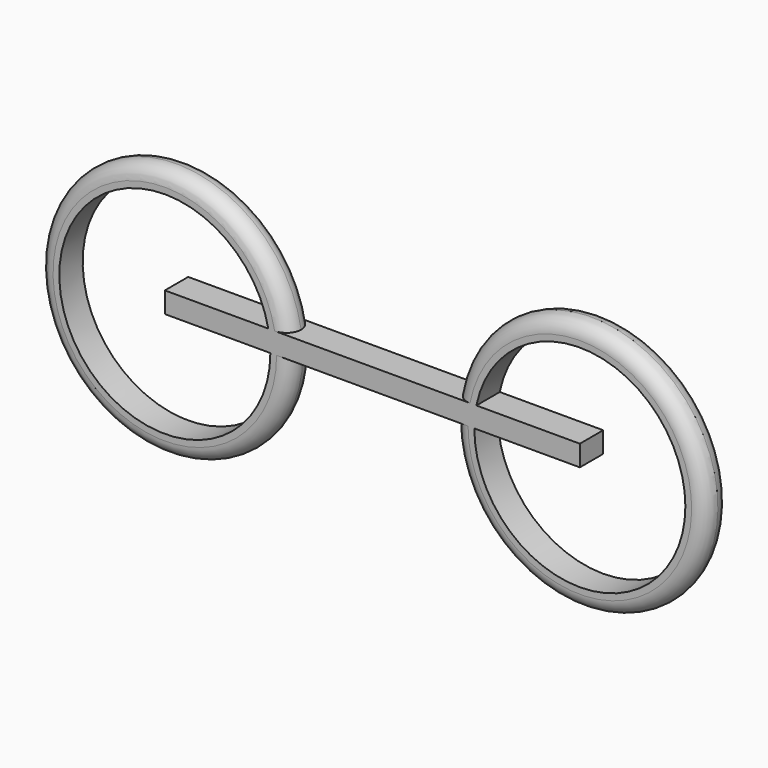
from build123d import *

# Parameters (mm, degrees)
F0_R     = 303
F0_R_2   = 253
F1_DEPTH = 70
F2_R     = 34.99999
F4_W     = 995
F4_H     = 50
F5_DEPTH = 70


# Not quite as in the source:
# - a fillet or chamfer is up to 0.001 mm smaller than in the source, because OpenCascade refuses the exact size


with BuildPart() as f1:
    # F0 (on Front) → F1 (new body)
    with BuildSketch(Plane.XZ):
        Circle(F0_R)
        Circle(F0_R_2, mode=Mode.SUBTRACT)
    extrude(amount=F1_DEPTH)

    # F2 (radius 35 in the source; OpenCascade refuses exactly that, so slightly less here)
    f2_edges = [f1.edges().sort_by_distance(p)[0] for p in [
        (-303, -70, 0),
        (-303, 0, 0),
    ]]
    fillet(f2_edges, radius=F2_R)


with BuildPart() as f3_1:
    # F3: copy of F1
    add(f1.part.moved(Location((995, 0, 0))))


with BuildPart() as f1_1:
    add(f1.part)

    add(f3_1.part)  # F5 merges F3_1
    # F4 (on Front) → F5 (join)
    with BuildSketch(Plane.XZ):
        with Locations((497.5, 25)):
            Rectangle(F4_W, F4_H)
    extrude(amount=F5_DEPTH)


solid = f1_1.part
